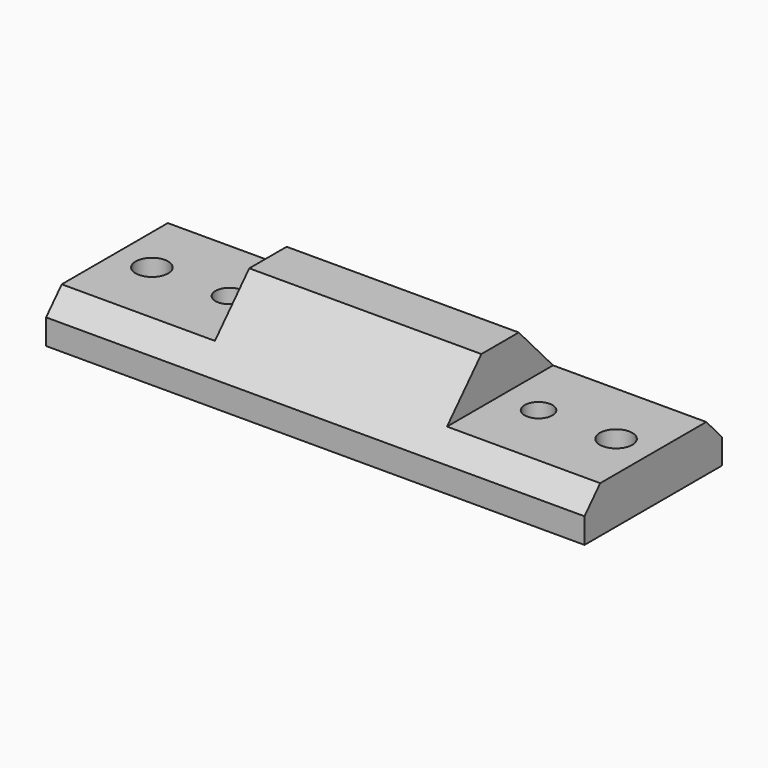
from build123d import *

# Parameters (mm, degrees)
F0_W          = 38
F0_H          = 18.5
F0_R          = 1.5
F0_W_2        = 10
F0_R_2        = 1.75
F1_DEPTH      = 10
F3_DEPTH      = 58.001
F4_W          = 16.5
F4_H          = 12
F5_DEPTH      = 25
F5_DEPTH_BACK = 25


with BuildPart() as f1:
    # F0 (on Top) → F1 (new body)
    with BuildSketch(Plane.XY):
        Rectangle(F0_W, F0_H)
        with Locations((-16.65, 0)):
            Circle(F0_R, mode=Mode.SUBTRACT)
        with Locations((16.65, 0)):
            Circle(F0_R, mode=Mode.SUBTRACT)
        with Locations((24, 0)):
            Rectangle(F0_W_2, F0_H)
        with Locations((25, 0)):
            Circle(F0_R_2, mode=Mode.SUBTRACT)
        with Locations((-24, 0)):
            Rectangle(F0_W_2, F0_H)
        with Locations((-25, 0)):
            Circle(F0_R_2, mode=Mode.SUBTRACT)
    extrude(amount=F1_DEPTH)

    # F2 (on face) → F3 (cut, through all)
    with BuildSketch(Plane.YZ.offset(29)):
        Polygon((-9.25, 10), (-9.25, 2.72), (-4.625, 7.72), (-2.516, 10), align=None)
        Polygon((2.516, 10), (4.625, 7.72), (9.25, 2.72), (9.25, 10), align=None)
    extrude(amount=-F3_DEPTH, mode=Mode.SUBTRACT)

    # F4 (on Front) → F5 (cut, two sides)
    with BuildSketch(Plane.XZ) as f5_sk:
        with Locations((-20.75, 11)):
            Rectangle(F4_W, F4_H)
        with Locations((20.75, 11)):
            Rectangle(F4_W, F4_H)
    extrude(amount=F5_DEPTH, mode=Mode.SUBTRACT)
    extrude(f5_sk.sketch, amount=-F5_DEPTH_BACK, mode=Mode.SUBTRACT)


solid = f1.part
